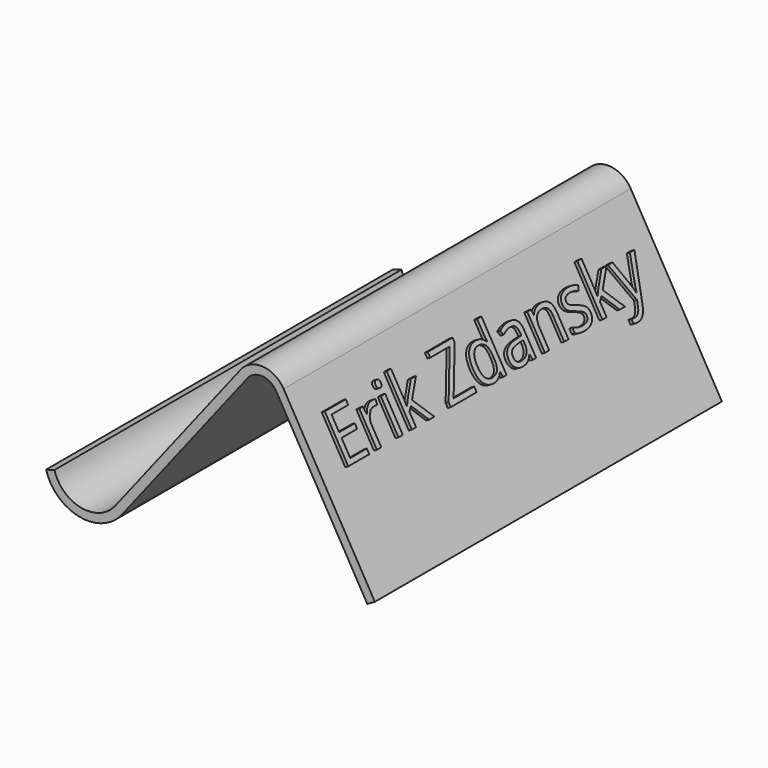
from build123d import *

# Parameters (mm, degrees)
F1_DEPTH     = 100
F2_TEXT_SIZE = 15.1894728515
F3_DEPTH     = 0.8


# Not quite as in the source:
# - Text() gives the source's letters only with a copy of the font that has no kerning and outlines rounded to 1/6400 em; it was checked with that copy


with BuildPart() as f1:
    # F0 (on Front) → F1 (new body)
    with BuildSketch(Plane.XZ):
        with BuildLine():
            Line((-5.4729582171, 37.0512587965), (-34.3901541668, 0))
            ThreePointArc((-34.3901541668, 0), (-42.2271285686, -2.9301814601), (-48.3901541668, 2.7285504329))
            Line((-48.3901541668, 2.7285504329), (-50.3135048564, 2.1801690646))
            ThreePointArc((-50.3135048564, 2.1801690646), (-42.6097228585, -4.8932458017), (-32.8135048564, -1.2305189766))
            Line((-32.8135048564, -1.2305189766), (-3.8963089066, 35.8207398199))
            ThreePointArc((-3.8963089066, 35.8207398199), (-0.4660195663, 37.3500998596), (2.7200708245, 35.3614683928))
            Line((2.7200708245, 35.3614683928), (23.7386193484, -1.000883263))
            Line((23.7386193484, -1.000883263), (25.4701599035, 0))
            Line((25.4701599035, 0), (4.4516113795, 36.3623516559))
            ThreePointArc((4.4516113795, 36.3623516559), (-0.3275242067, 39.345298856), (-5.4729582171, 37.0512587965))
        make_face()
    extrude(amount=F1_DEPTH)

    # F2 (on face) → F3 (join)
    with BuildSketch(Plane(origin=(19.0913665344, 0, 11.0353922565), x_dir=(0, 1, 0), z_dir=(0.8657702775, 0, 0.5004416315))):
        with Locations((-95, 11.2476888622)):
            Text('Erik Zdansky', F2_TEXT_SIZE, font='Open Sans', text_align=(TextAlign.LEFT, TextAlign.BOTTOM))
    extrude(amount=F3_DEPTH)


solid = f1.part
